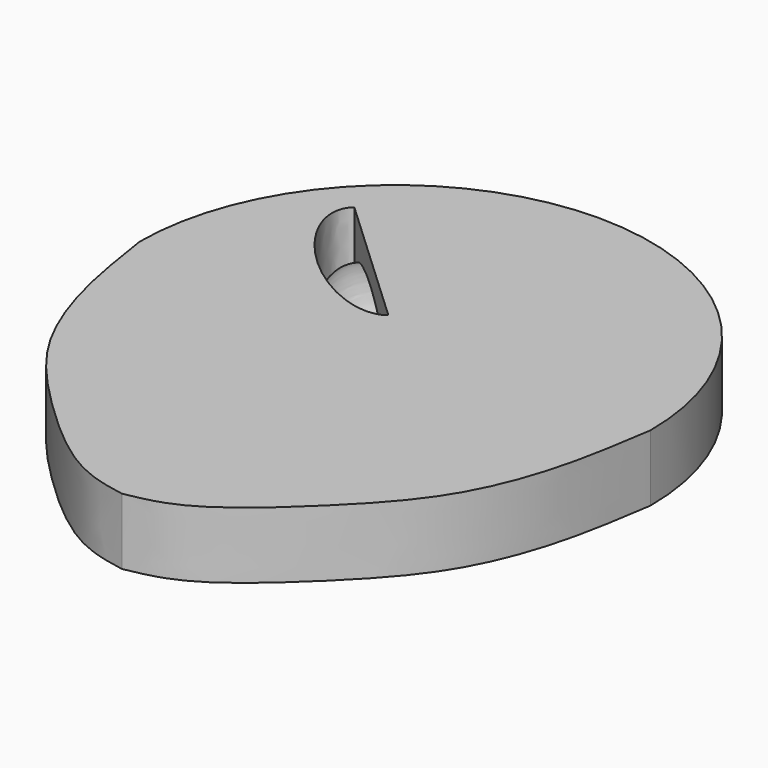
from build123d import *

# Parameters (mm, degrees)
F3_DEPTH = 25.4


with BuildPart() as f1:
    # F0 (on Top) → F1 (revolve)
    with BuildSketch(Plane.XY):
        with BuildLine():
            Line((-9.9525216629, 9.2959710391), (-61.5633883725, 57.502158223))
            add(Edge.make_bspline(
                [(-61.5633883725, 57.502158223), (-74.2319049125, 47.3361252787), (-48.4264715577, 23.2330316867), (-22.6210382029, -0.8700619052), (-9.9525216629, 9.2959710391)],
                knots=[6.2006468794, 6.2006468794, 6.2006468794, 7.7714432062, 7.7714432062, 9.342239533, 9.342239533, 9.342239533], degree=2, weights=[1, 0.7071067812, 1, 0.7071067812, 1]))
        make_face()
    revolve(axis=Axis((-35.7579550177, 33.399064631, 0), (-0.7308006287, 0.6825909764, 0)))


with BuildPart() as f2_1:
    # F2: instance of F1
    add(f1.part.mirror(Plane.YZ))


with BuildPart() as f3:
    # F0 (on Top) → F3 (new body)
    with BuildSketch(Plane.XY):
        with BuildLine():
            Line((0, 0), (0, 97.8596722921))
            ThreePointArc((0, 97.8596722921), (-38.9850767718, 89.7590065131), (-71.5159100355, 66.7981292621))
            Line((-71.5159100355, 66.7981292621), (-61.5633883725, 57.502158223))
            Line((-61.5633883725, 57.502158223), (-9.9525216629, 9.2959710391))
            Line((-9.9525216629, 9.2959710391), (0, 0))
        make_face()
        with BuildLine():
            ThreePointArc((97.8596722921, 0), (69.1972378824, 69.1972378824), (0, 97.8596722921))
            Line((0, 97.8596722921), (0, 0))
            Line((0, 0), (0, -130.7861357927))
            add(Edge.make_bspline(
                [(97.8596722921, 0), (96.0268468146, -11.9272951744), (92.5053784341, -35.7053882501), (79.3134540192, -70.0190893438), (55.4290042275, -96.7287402044), (22.4434714007, -126.5741021306), (6.5719517026, -129.5530993253), (0, -130.7861357927)],
                knots=[0, 0, 0, 0, 0.2054206984, 0.4088183981, 0.616122195, 0.8410568868, 1, 1, 1, 1], degree=3))
        make_face()
        with BuildLine():
            Line((-61.5633883725, 57.502158223), (-71.5159100355, 66.7981292621))
            ThreePointArc((-71.5159100355, 66.7981292621), (-91.0358143284, 35.9025900276), (-97.8596722921, 0))
            Line((-97.8596722921, 0), (0, 0))
            Line((0, 0), (-9.9525216629, 9.2959710391))
            add(Edge.make_bspline(
                [(-61.5633883725, 57.502158223), (-74.2319049125, 47.3361252787), (-48.4264715577, 23.2330316867), (-22.6210382029, -0.8700619052), (-9.9525216629, 9.2959710391)],
                knots=[6.2006468794, 6.2006468794, 6.2006468794, 7.7714432062, 7.7714432062, 9.342239533, 9.342239533, 9.342239533], degree=2, weights=[1, 0.7071067812, 1, 0.7071067812, 1]))
        make_face()
        with BuildLine():
            Line((0, -130.7861357927), (0, 0))
            Line((0, 0), (-97.8596722921, 0))
            add(Edge.make_bspline(
                [(-97.8596722921, 0), (-96.0268468146, -11.9272951744), (-92.5053784341, -35.7053882501), (-79.3134540192, -70.0190893438), (-55.4290042275, -96.7287402044), (-22.4434714007, -126.5741021306), (-6.5719517026, -129.5530993253), (0, -130.7861357927)],
                knots=[0, 0, 0, 0, 0.2054206984, 0.4088183981, 0.616122195, 0.8410568868, 1, 1, 1, 1], degree=3))
        make_face()
    extrude(amount=F3_DEPTH)


solid = Compound([f1.part, f2_1.part, f3.part])
